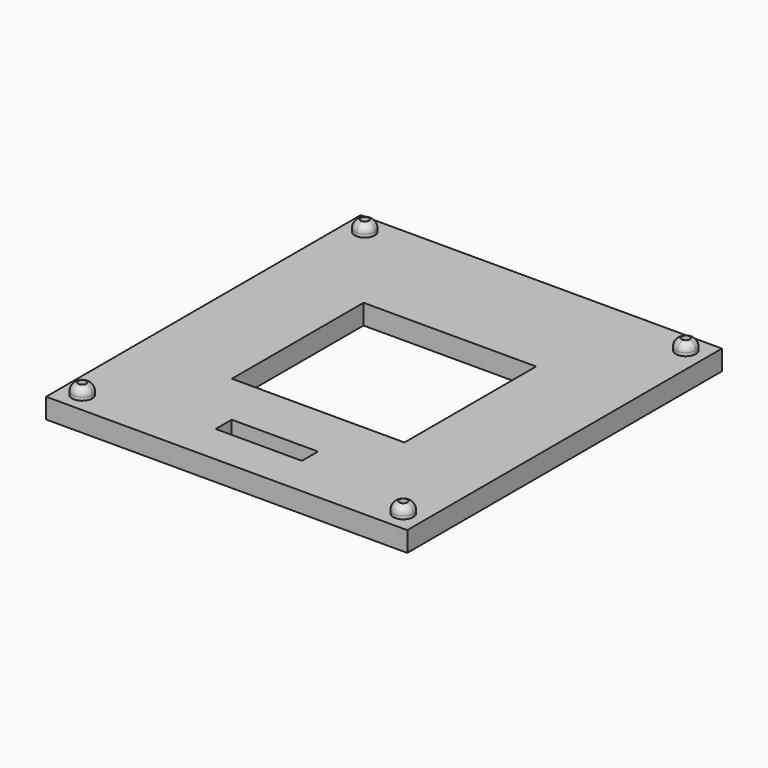
from build123d import *

# Parameters (mm, degrees)
F1_DEPTH = 5
F0_W     = 90
F0_H     = 98
F2_DEPTH = 5
F3_DEPTH = 7.8
F4_R     = 2
F5_D     = 2
F6_R     = 1


with BuildPart() as f1:
    # F0 (on Top) → F1 (new body)
    with BuildSketch(Plane.XY):
        Polygon((43.3765034378, 40.0858414471), (-26.6234965622, 40.0858414471), (-26.6234965622, -37.9141585529), (-2.3734965622, -37.9141585529), (-2.3734965622, -32.9141585529), (19.1265034378, -32.9141585529), (19.1265034378, -37.9141585529), (43.3765034378, -37.9141585529), align=None)
        Polygon((29.8765034378, -15.1862744242), (29.8765034378, -19.4141585529), (25.4069790244, -19.4141585529), (-8.9896805584, -19.4141585529), (-13.1234965622, -19.4141585529), (-13.1234965622, -15.039251186), (-13.1234965622, 18.1580353528), (-13.1234965622, 21.5858414471), (-9.5030404627, 21.5858414471), (25.7939789444, 21.5858414471), (29.8765034378, 21.5858414471), (29.8765034378, 17.3397138715), align=None, mode=Mode.SUBTRACT)
    extrude(amount=F1_DEPTH)

    # F0 (on Top) → F2 (join)
    with BuildSketch(Plane.XY):
        with Locations((8.3765034378, 1.0858414471)):
            Rectangle(F0_W, F0_H)
        with BuildLine():
            ThreePointArc((-31.6234965622, 42.5858414471), (-33.3912635152, 46.8536084001), (-29.1234965622, 45.0858414471))
            Line((-29.1234965622, 45.0858414471), (45.8765034378, 45.0858414471))
            ThreePointArc((45.8765034378, 45.0858414471), (48.3765034378, 47.5858414471), (50.8765034378, 45.0858414471))
            ThreePointArc((50.8765034378, 45.0858414471), (50.1442703907, 43.3180744941), (48.3765034378, 42.5858414471))
            Line((48.3765034378, 42.5858414471), (48.3765034378, -40.4141585529))
            ThreePointArc((48.3765034378, -40.4141585529), (50.1442703907, -41.1463915999), (50.8765034378, -42.9141585529))
            ThreePointArc((50.8765034378, -42.9141585529), (48.3765034378, -45.4141585529), (45.8765034378, -42.9141585529))
            Line((45.8765034378, -42.9141585529), (-29.1234965622, -42.9141585529))
            ThreePointArc((-29.1234965622, -42.9141585529), (-33.3912635152, -44.6819255059), (-31.6234965622, -40.4141585529))
            Line((-31.6234965622, -40.4141585529), (-31.6234965622, 42.5858414471))
        make_face(mode=Mode.SUBTRACT)
        with BuildLine():
            Line((45.8765034378, 45.0858414471), (-29.1234965622, 45.0858414471))
            ThreePointArc((-29.1234965622, 45.0858414471), (-29.8557296093, 43.3180744941), (-31.6234965622, 42.5858414471))
            Line((-31.6234965622, 42.5858414471), (-31.6234965622, -40.4141585529))
            ThreePointArc((-31.6234965622, -40.4141585529), (-29.8557296093, -41.1463915999), (-29.1234965622, -42.9141585529))
            Line((-29.1234965622, -42.9141585529), (45.8765034378, -42.9141585529))
            ThreePointArc((45.8765034378, -42.9141585529), (46.6087364848, -41.1463915999), (48.3765034378, -40.4141585529))
            Line((48.3765034378, -40.4141585529), (48.3765034378, 42.5858414471))
            ThreePointArc((48.3765034378, 42.5858414471), (46.6087364848, 43.3180744941), (45.8765034378, 45.0858414471))
        make_face()
        Polygon((-26.6234965622, -37.9141585529), (-26.6234965622, 40.0858414471), (43.3765034378, 40.0858414471), (43.3765034378, -37.9141585529), (19.1265034378, -37.9141585529), (-2.3734965622, -37.9141585529), align=None, mode=Mode.SUBTRACT)
    extrude(amount=F2_DEPTH)

    # F0 (on Top) → F3 (join)
    with BuildSketch(Plane.XY):
        with BuildLine():
            Line((-31.6234965622, 42.5858414471), (-31.6234965622, 45.0858414471))
            Line((-31.6234965622, 45.0858414471), (-29.1234965622, 45.0858414471))
            ThreePointArc((-29.1234965622, 45.0858414471), (-33.3912635152, 46.8536084001), (-31.6234965622, 42.5858414471))
        make_face()
        with BuildLine():
            Line((-29.1234965622, 45.0858414471), (-31.6234965622, 45.0858414471))
            Line((-31.6234965622, 45.0858414471), (-31.6234965622, 42.5858414471))
            ThreePointArc((-31.6234965622, 42.5858414471), (-29.8557296093, 43.3180744941), (-29.1234965622, 45.0858414471))
        make_face()
        with BuildLine():
            Line((48.3765034378, 45.0858414471), (45.8765034378, 45.0858414471))
            ThreePointArc((45.8765034378, 45.0858414471), (46.6087364848, 43.3180744941), (48.3765034378, 42.5858414471))
            Line((48.3765034378, 42.5858414471), (48.3765034378, 45.0858414471))
        make_face()
        with BuildLine():
            ThreePointArc((50.8765034378, 45.0858414471), (48.3765034378, 47.5858414471), (45.8765034378, 45.0858414471))
            Line((45.8765034378, 45.0858414471), (48.3765034378, 45.0858414471))
            Line((48.3765034378, 45.0858414471), (48.3765034378, 42.5858414471))
            ThreePointArc((48.3765034378, 42.5858414471), (50.1442703907, 43.3180744941), (50.8765034378, 45.0858414471))
        make_face()
        with BuildLine():
            ThreePointArc((50.8765034378, -42.9141585529), (50.1442703907, -41.1463915999), (48.3765034378, -40.4141585529))
            Line((48.3765034378, -40.4141585529), (48.3765034378, -42.9141585529))
            Line((48.3765034378, -42.9141585529), (45.8765034378, -42.9141585529))
            ThreePointArc((45.8765034378, -42.9141585529), (48.3765034378, -45.4141585529), (50.8765034378, -42.9141585529))
        make_face()
        with BuildLine():
            Line((48.3765034378, -42.9141585529), (48.3765034378, -40.4141585529))
            ThreePointArc((48.3765034378, -40.4141585529), (46.6087364848, -41.1463915999), (45.8765034378, -42.9141585529))
            Line((45.8765034378, -42.9141585529), (48.3765034378, -42.9141585529))
        make_face()
        with BuildLine():
            Line((-31.6234965622, -42.9141585529), (-31.6234965622, -40.4141585529))
            ThreePointArc((-31.6234965622, -40.4141585529), (-33.3912635152, -44.6819255059), (-29.1234965622, -42.9141585529))
            Line((-29.1234965622, -42.9141585529), (-31.6234965622, -42.9141585529))
        make_face()
        with BuildLine():
            ThreePointArc((-29.1234965622, -42.9141585529), (-29.8557296093, -41.1463915999), (-31.6234965622, -40.4141585529))
            Line((-31.6234965622, -40.4141585529), (-31.6234965622, -42.9141585529))
            Line((-31.6234965622, -42.9141585529), (-29.1234965622, -42.9141585529))
        make_face()
    extrude(amount=F3_DEPTH)

    # F4
    f4_edges = [f1.edges().sort_by_distance(p)[0] for p in [
        (-31.623497, 47.585841, 7.8),
        (-34.123497, -42.914159, 7.8),
        (48.376503, -45.414159, 7.8),
        (48.376503, 47.585841, 7.8),
    ]]
    fillet(f4_edges, radius=F4_R)

    # F5 (through all)
    with Locations(Plane(origin=(0, 0, 0), x_dir=(1, 0, 0), z_dir=(0, 0, -1))):
        with Locations((48.3765034378, -45.0858414471), (48.3765034378, 42.9141585529), (-31.6234965622, 42.9141585529), (-31.6234965622, -45.0858414471)):
            Hole(F5_D / 2)

    # F6
    f6_edges = [f1.edges().sort_by_distance(p)[0] for p in [
        (8.376503, -32.914159, 0),
    ]]
    fillet(f6_edges, radius=F6_R)


solid = f1.part
